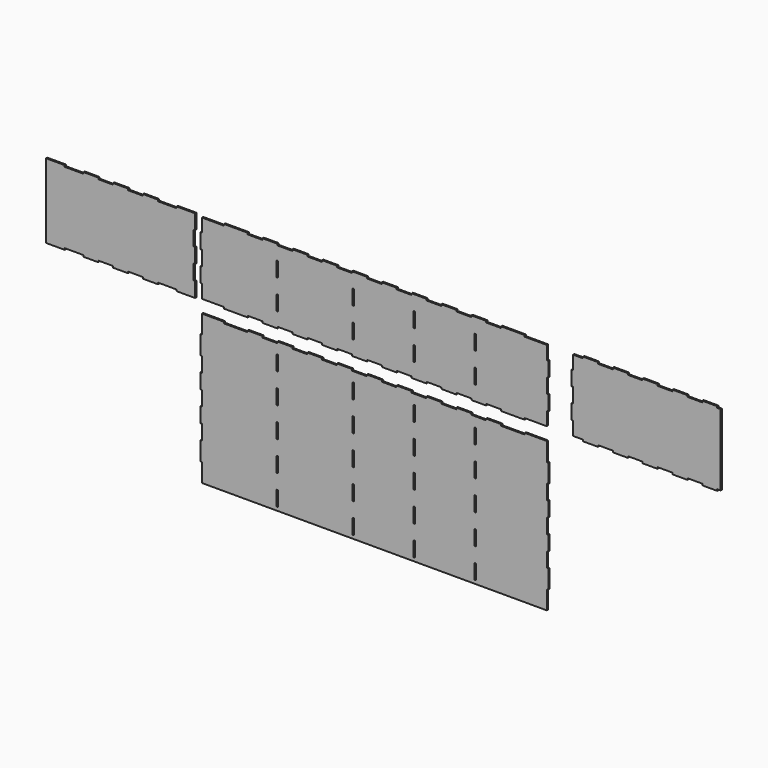
from build123d import *

# Parameters (mm, degrees)
F1_DEPTH = 3
F2_W     = 604.999964
F2_H     = 3.000021
F3_DEPTH = 3
F4_W     = 3
F4_H     = 89.999995
F5_DEPTH = 3
F7_DEPTH = 3
F8_W     = 3
F8_H     = 29.999999
F8_H_2   = 30.000003
F9_DEPTH = 3.001


# Not quite as in the source:
# - ends of sketch curves that miss each other by under 0.0002 mm in the source are joined


with BuildPart() as f1:
    # F0 (on Front) → F1 (new body)
    with BuildSketch(Plane.XZ):
        Polygon((-505.292158, 116.601969), (-505.292158, 86.60197), (-467.792159, 86.60197), (-467.792159, 89.60197), (-430.292159, 89.60197), (-430.292159, 86.60197), (-400.292165, 86.60197), (-400.292165, 89.60197), (-370.292162, 89.60197), (-370.292162, 86.60197), (-340.292159, 86.60197), (-340.292159, 89.60197), (-310.292173, 89.60197), (-310.292173, 86.60197), (-280.29217, 86.60197), (-280.29217, 89.60197), (-242.792167, 89.60197), (-242.792167, 86.60197), (-205.292163, 86.60197), (-205.292163, 116.601969), (-208.292184, 116.601969), (-208.292184, 146.601967), (-205.292163, 146.601967), (-205.292163, 176.601961), (-208.292184, 176.601961), (-208.292184, 206.601964), (-205.292163, 206.601964), (-205.292163, 236.601967), (-242.792167, 236.601967), (-242.792167, 233.601964), (-280.29217, 233.601964), (-280.29217, 236.601967), (-310.292173, 236.601967), (-310.292173, 233.601964), (-340.292159, 233.601964), (-340.292159, 236.601967), (-370.292162, 236.601967), (-370.292162, 233.601964), (-400.292165, 233.601964), (-400.292165, 236.601967), (-430.292159, 236.601967), (-430.292159, 233.601964), (-467.792159, 233.601964), (-467.792159, 236.601967), (-505.292158, 236.601967), (-505.292158, 206.601964), (-502.292158, 206.601964), (-502.292158, 176.601961), (-505.292158, 176.601961), (-505.292158, 146.601967), (-502.292158, 146.601967), (-502.292158, 116.601969), align=None)
    extrude(amount=F1_DEPTH)

    # F4 (on face) → F5 (join)
    with BuildSketch(Plane.XZ.offset(3)):
        with Locations((-503.792158, 161.6019665)):
            Rectangle(F4_W, F4_H)
    extrude(amount=-F5_DEPTH)


with BuildPart() as f1b:
    # F0 (on Front) → F1, piece 2 (new body)
    with BuildSketch(Plane.XZ):
        Polygon((-147.207775, 63.398028), (-191.707772, 63.398028), (-191.707772, 25.898029), (-194.707771, 25.898029), (-194.707771, -11.60197), (-191.707772, -11.60197), (-191.707772, -41.601965), (-194.707771, -41.601965), (-194.707771, -71.601968), (-191.707772, -71.601968), (-191.707772, -101.601971), (-194.707771, -101.601971), (-194.707771, -131.601956), (-191.707772, -131.601956), (-191.707772, -161.601959), (-194.707771, -161.601959), (-194.707771, -199.101963), (-191.707772, -199.101963), (-191.707772, -236.601967), (-147.207775, -236.601967), (-147.207775, -233.601946), (-99.707779, -233.601946), (-99.707779, -236.601967), (-69.707776, -236.601967), (-69.707776, -233.601946), (-39.707774, -233.601946), (-39.707774, -236.601967), (-9.707788, -236.601967), (-9.707788, -233.601946), (20.292215, -233.601946), (20.292215, -236.601967), (50.292218, -236.601967), (50.292218, -233.601946), (80.292221, -233.601946), (80.292221, -236.601967), (110.292224, -236.601967), (110.292224, -233.601946), (140.292192, -233.601946), (140.292192, -236.601967), (170.292195, -236.601967), (170.292195, -233.601946), (200.292198, -233.601946), (200.292198, -236.601967), (230.292201, -236.601967), (230.292201, -233.601946), (260.292204, -233.601946), (260.292204, -236.601967), (290.292207, -236.601967), (290.292207, -233.601946), (320.29221, -233.601946), (320.29221, -236.601967), (350.292213, -236.601967), (350.292213, -233.601946), (380.292181, -233.601946), (380.292181, -236.601967), (410.292218, -236.601967), (410.292218, -233.601946), (457.792189, -233.601946), (457.792189, -236.601967), (502.292172, -236.601967), (502.292172, -199.101963), (505.292159, -199.101963), (505.292159, -161.601959), (502.292172, -161.601959), (502.292172, -131.601956), (505.292159, -131.601956), (505.292159, -101.601971), (502.292172, -101.601971), (502.292172, -71.601968), (505.292159, -71.601968), (505.292159, -41.601965), (502.292172, -41.601965), (502.292172, -11.60197), (505.292159, -11.60197), (505.292159, 25.898029), (502.292172, 25.898029), (502.292172, 63.398028), (457.792189, 63.398028), (457.792189, 60.398028), (410.292218, 60.398028), (410.292218, 63.398028), (380.292181, 63.398028), (380.292181, 60.398028), (350.292213, 60.398028), (350.292213, 63.398028), (320.29221, 63.398028), (320.29221, 60.398028), (290.292207, 60.398028), (290.292207, 63.398028), (260.292204, 63.398028), (260.292204, 60.398028), (230.292201, 60.398028), (230.292201, 63.398028), (200.292198, 63.398028), (200.292198, 60.398028), (170.292195, 60.398028), (170.292195, 63.398028), (140.292192, 63.398028), (140.292192, 60.398028), (110.292224, 60.398028), (110.292224, 63.398028), (80.292221, 63.398028), (80.292221, 60.398028), (50.292218, 60.398028), (50.292218, 63.398028), (20.292215, 63.398028), (20.292215, 60.398028), (-9.707788, 60.398028), (-9.707788, 63.398028), (-39.707774, 63.398028), (-39.707774, 60.398028), (-69.707776, 60.398028), (-69.707776, 63.398028), (-99.707779, 63.398028), (-99.707779, 60.398028), (-147.207775, 60.398028), align=None)
    extrude(amount=F1_DEPTH)

    # F2 (on face) → F3 (join)
    with BuildSketch(Plane.XZ.offset(3)):
        with Locations((155.292207, -235.1019565)):
            Rectangle(F2_W, F2_H)
    extrude(amount=-F3_DEPTH)


with BuildPart() as f1c:
    # F0 (on Front) → F1, piece 3 (new body)
    with BuildSketch(Plane.XZ):
        Polygon((502.292159, 206.601969), (502.292159, 233.601968), (457.792163, 233.601968), (457.792163, 236.601967), (410.292167, 236.601967), (410.292167, 233.601968), (380.292164, 233.601968), (380.292164, 236.601967), (350.292161, 236.601967), (350.292161, 233.601968), (320.292175, 233.601968), (320.292175, 236.601967), (290.292172, 236.601967), (290.292172, 233.601968), (260.292169, 233.601968), (260.292169, 236.601967), (230.292167, 236.601967), (230.292167, 233.601968), (200.292164, 233.601968), (200.292164, 236.601967), (170.292195, 236.601967), (170.292195, 233.601968), (140.292192, 233.601968), (140.292192, 236.601967), (110.292189, 236.601967), (110.292189, 233.601968), (80.292186, 233.601968), (80.292186, 236.601967), (50.292184, 236.601967), (50.292184, 233.601968), (20.292181, 233.601968), (20.292181, 236.601967), (-9.707822, 236.601967), (-9.707822, 233.601968), (-39.707825, 233.601968), (-39.707825, 236.601967), (-69.707794, 236.601967), (-69.707794, 233.601968), (-99.707831, 233.601968), (-99.707831, 236.601967), (-147.207801, 236.601967), (-147.207801, 233.601968), (-191.707785, 233.601968), (-191.707785, 206.601969), (-194.707771, 206.601969), (-194.707771, 176.60197), (-191.707785, 176.60197), (-191.707785, 146.601976), (-194.707771, 146.601976), (-194.707771, 116.601973), (-191.707785, 116.601973), (-191.707785, 89.601974), (-147.207801, 89.601974), (-147.207801, 86.60197), (-99.707831, 86.60197), (-99.707831, 89.601974), (-69.707794, 89.601974), (-69.707794, 86.60197), (-39.707825, 86.60197), (-39.707825, 89.601974), (-9.707822, 89.601974), (-9.707822, 86.60197), (20.292181, 86.60197), (20.292181, 89.601974), (50.292184, 89.601974), (50.292184, 86.60197), (80.292186, 86.60197), (80.292186, 89.601974), (110.292189, 89.601974), (110.292189, 86.60197), (140.292192, 86.60197), (140.292192, 89.601974), (170.292195, 89.601974), (170.292195, 86.60197), (200.292164, 86.60197), (200.292164, 89.601974), (230.292167, 89.601974), (230.292167, 86.60197), (260.292169, 86.60197), (260.292169, 89.601974), (290.292172, 89.601974), (290.292172, 86.60197), (320.292175, 86.60197), (320.292175, 89.601974), (350.292161, 89.601974), (350.292161, 86.60197), (380.292164, 86.60197), (380.292164, 89.601974), (410.292167, 89.601974), (410.292167, 86.60197), (457.792163, 86.60197), (457.792163, 89.601974), (502.292159, 89.601974), (502.292159, 116.601973), (505.292159, 116.601973), (505.292159, 146.601976), (502.292159, 146.601976), (502.292159, 176.60197), (505.292159, 176.60197), (505.292159, 206.601969), align=None)
    extrude(amount=F1_DEPTH)


with BuildPart() as f7:
    # F6 (on face) → F7 (new body)
    with BuildSketch(Plane.XZ.offset(3)):
        Polygon((575.274784565, 233.601968), (555.274784565, 233.601968), (555.274784565, 206.601969), (552.274784565, 206.601969), (552.274784565, 176.60197), (555.274784565, 176.60197), (555.274784565, 146.601976), (552.274784565, 146.601976), (552.274784565, 116.601973), (555.274784565, 116.601973), (555.274784565, 89.601974), (575.274784565, 89.601978), (575.274784565, 86.601978), (605.274783565, 86.601978), (605.274783565, 89.601978), (635.274784565, 89.601978), (635.274784565, 86.601978), (665.274783565, 86.601978), (665.274783565, 89.601978), (695.274784565, 89.601978), (695.274784565, 86.601978), (725.274783565, 86.601978), (725.274783565, 89.601978), (755.274784565, 89.601978), (755.274784565, 86.601978), (785.274783565, 86.601978), (785.274783565, 89.601978), (815.274784565, 89.601978), (815.274784565, 86.601978), (845.274783565, 86.601978), (845.274783565, 89.601978), (852.274758565, 89.601978), (852.274758565, 233.601968), (845.274783565, 233.601968), (845.274783565, 236.601968), (815.274784565, 236.601968), (815.274784565, 233.601968), (785.274783565, 233.601968), (785.274783565, 236.601968), (755.274784565, 236.601968), (755.274784565, 233.601968), (725.274783565, 233.601968), (725.274783565, 236.601968), (695.274784565, 236.601968), (695.274784565, 233.601968), (665.274783565, 233.601968), (665.274783565, 236.601968), (635.274784565, 236.601968), (635.274784565, 233.601968), (605.274783565, 233.601968), (605.274783565, 236.601968), (575.274784565, 236.601968), align=None)
    extrude(amount=-F7_DEPTH)


with BuildPart() as f9_tool:
    # F8 (on face) → F9 (new body, through all)
    with BuildSketch(Plane.XZ.offset(3)):
        with Locations((-40.207785, 191.6019695)):
            Rectangle(F8_W, F8_H)
        with Locations((-40.207785, 131.6019745)):
            Rectangle(F8_W, F8_H_2)
        with Locations((-40.207785, 25.3980285)):
            Rectangle(F8_W, F8_H)
        with Locations((-40.207785, -34.6019715)):
            Rectangle(F8_W, F8_H)
        with Locations((-40.207785, -94.6019715)):
            Rectangle(F8_W, F8_H)
        with Locations((-40.207785, -154.6019715)):
            Rectangle(F8_W, F8_H)
        with Locations((-40.207785, -214.6019715)):
            Rectangle(F8_W, F8_H)
        with Locations((112.792215, -214.6019715)):
            Rectangle(F8_W, F8_H)
        with Locations((112.792215, -94.6019715)):
            Rectangle(F8_W, F8_H)
        with Locations((112.792215, -34.6019715)):
            Rectangle(F8_W, F8_H)
        with Locations((112.792215, 25.3980285)):
            Rectangle(F8_W, F8_H)
        with Locations((112.792215, -154.6019715)):
            Rectangle(F8_W, F8_H)
        with Locations((112.792215, 131.6019745)):
            Rectangle(F8_W, F8_H_2)
        with Locations((112.792215, 191.6019695)):
            Rectangle(F8_W, F8_H)
        with Locations((235.792215, -154.6019715)):
            Rectangle(F8_W, F8_H)
        with Locations((235.792215, -214.6019715)):
            Rectangle(F8_W, F8_H)
        with Locations((235.792215, -34.6019715)):
            Rectangle(F8_W, F8_H)
        with Locations((235.792215, -94.6019715)):
            Rectangle(F8_W, F8_H)
        with Locations((235.792215, 25.3980285)):
            Rectangle(F8_W, F8_H)
        with Locations((358.792215, -94.6019715)):
            Rectangle(F8_W, F8_H)
        with Locations((358.792215, -154.6019715)):
            Rectangle(F8_W, F8_H)
        with Locations((358.792215, -34.6019715)):
            Rectangle(F8_W, F8_H)
        with Locations((358.792215, -214.6019715)):
            Rectangle(F8_W, F8_H)
        with Locations((358.792215, 25.3980285)):
            Rectangle(F8_W, F8_H)
        with Locations((235.792215, 191.6019695)):
            Rectangle(F8_W, F8_H)
        with Locations((235.792215, 131.6019745)):
            Rectangle(F8_W, F8_H_2)
        with Locations((358.792215, 131.6019745)):
            Rectangle(F8_W, F8_H_2)
        with Locations((358.792215, 191.6019695)):
            Rectangle(F8_W, F8_H)
    extrude(amount=-F9_DEPTH)


with BuildPart() as f1b_1:
    add(f1b.part)

    # F9: cut by f9_tool
    add(f9_tool.part, mode=Mode.SUBTRACT)


with BuildPart() as f1c_1:
    add(f1c.part)

    # F9: cut by f9_tool
    add(f9_tool.part, mode=Mode.SUBTRACT)


solid = Compound([f1.part, f7.part, f1b_1.part, f1c_1.part])
